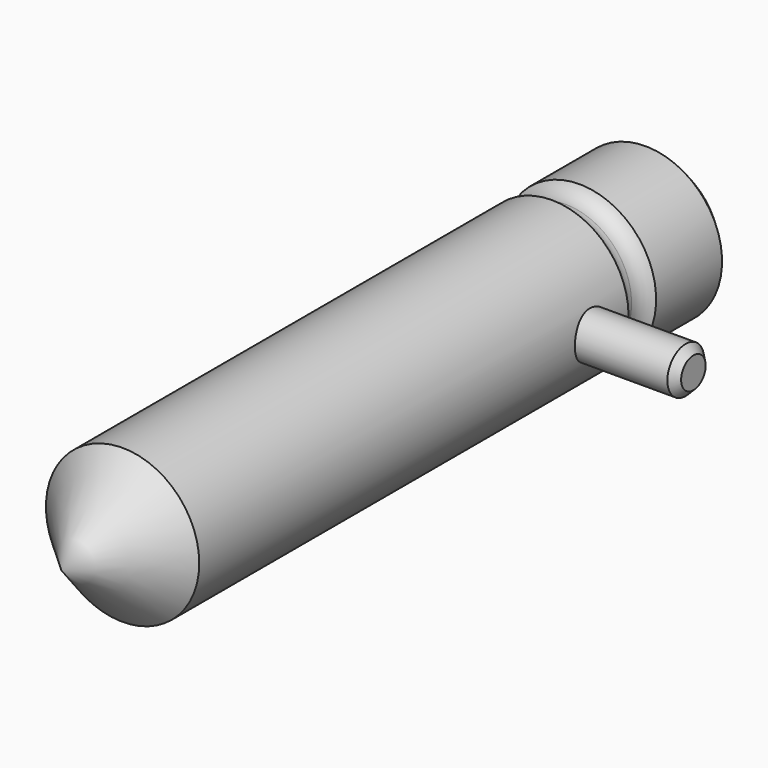
from build123d import *

# Parameters (mm, degrees)
F0_R     = 5
F1_DEPTH = 40
F2_R     = 4.3
F3_DEPTH = 2.25
F4_R     = 5
F5_DEPTH = 6.375
F7_SIZE  = 1
F8_R     = 1.5
F9_DEPTH = 11.53
F10_SIZE = 0.5
F11_SIZE = 5


# Not quite as in the source:
# - a fillet or chamfer that OpenCascade refuses, or shapes differently, is made with other operations: its cross-section is extruded or revolved along the edge and cut away or added


with BuildPart() as f1:
    # F0 (on Front) → F1 (new body)
    with BuildSketch(Plane.XZ):
        Circle(F0_R)
    extrude(amount=F1_DEPTH)

    # F2 (on face) → F3 (join)
    with BuildSketch(Plane(origin=(0, 0, 0), x_dir=(-1, 0, 0), z_dir=(0, 1, 0))):
        Circle(F2_R)
    extrude(amount=F3_DEPTH)

    # F4 (on face) → F5 (join)
    with BuildSketch(Plane(origin=(0, 2.25, 0), x_dir=(-1, 0, 0), z_dir=(0, 1, 0))):
        Circle(F4_R)
    extrude(amount=F5_DEPTH)

    # F6: fillet of radius 1.25 on 3 edges, made by hand

    # F6_s1 → F6_t2 (revolve)
    with BuildSketch(Plane.XY):
        with BuildLine():
            ThreePointArc((-4.3, 1.122497216), (-4.4893398282, 0.4610593883), (-5, 0))
            Line((-5, 0), (-4.3, 0))
            Line((-4.3, 0), (-4.3, 1.122497216))
        make_face()
    revolve(axis=Axis((0, 0, 0), (0, 1, 0)))

    # F6_s3 → F6_t4 (revolve)
    with BuildSketch(Plane.XY):
        with BuildLine():
            ThreePointArc((-5, 2.25), (-4.4893398282, 1.7889406117), (-4.3, 1.127502784))
            Line((-4.3, 1.127502784), (-4.3, 2.25))
            Line((-4.3, 2.25), (-5, 2.25))
        make_face()
    revolve(axis=Axis((0, 2.25, 0), (0, 1, 0)))

    # F7
    f7_edges = [f1.edges().sort_by_distance(p)[0] for p in [
        (5, 8.625, 0),
    ]]
    chamfer(f7_edges, length=F7_SIZE)

    # F8 (on Right) → F9 (join)
    with BuildSketch(Plane.YZ):
        with Locations((-2.875, 0)):
            Circle(F8_R)
    extrude(amount=F9_DEPTH)

    # F10
    f10_edges = [f1.edges().sort_by_distance(p)[0] for p in [
        (11.53, -4.375, 0),
    ]]
    chamfer(f10_edges, length=F10_SIZE)

    # F11
    f11_edges = [f1.edges().sort_by_distance(p)[0] for p in [
        (-5, -40, 0),
    ]]
    chamfer(f11_edges, length=F11_SIZE)


solid = f1.part
